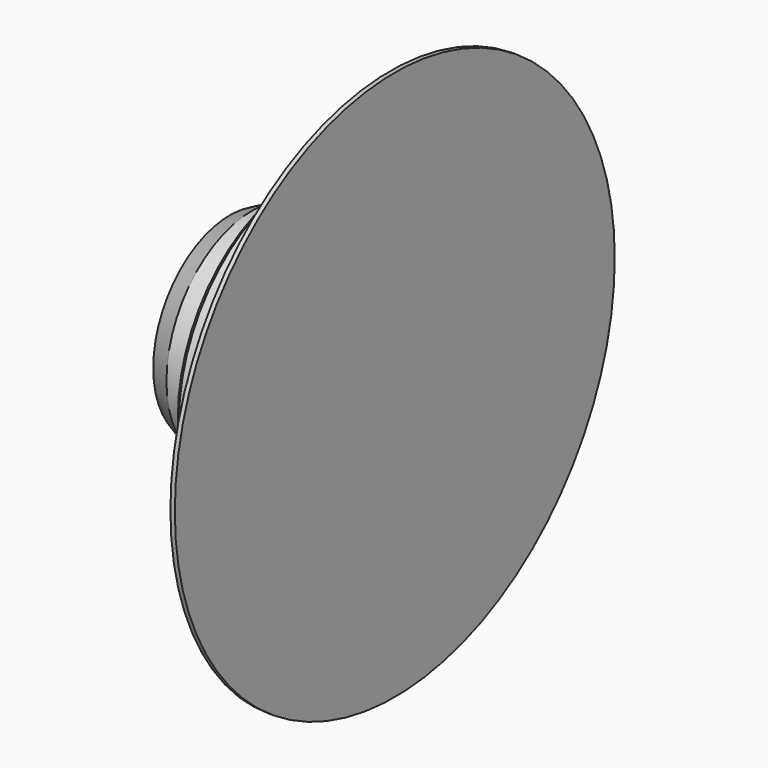
from build123d import *

# Parameters (mm, degrees)
F0_R       = 10
F1_DEPTH   = 4
F2_R       = 4.85
F3_DEPTH   = 3.5
F4_R       = 6.95
F4_R_2     = 6
F5_DEPTH   = 0.5
F6_R       = 10
F6_R_2     = 6.95
F7_DEPTH   = 3
F8_SIZE    = 0.25
F9_SIZE2   = 0.99999
F9_SIZE    = 0.49999
F9_2_SIZE2 = 1
F9_2_SIZE  = 0.5
F10_R      = 12.5
F10_R_2    = 9.5
F11_DEPTH  = 0.2


# Not quite as in the source:
# - a fillet or chamfer is up to 0.001 mm smaller than in the source, because OpenCascade refuses the exact size


with BuildPart() as f1:
    # F0 (on Right) → F1 (new body)
    with BuildSketch(Plane.YZ):
        Circle(F0_R)
    extrude(amount=F1_DEPTH)

    # F2 (on face) → F3 (join)
    with BuildSketch(Plane(origin=(0, 0, 0), x_dir=(0, -1, 0), z_dir=(-1, 0, 0))):
        Circle(F2_R)
    extrude(amount=F3_DEPTH)

    # F4 (on face) → F5 (join)
    with BuildSketch(Plane(origin=(0, 0, 0), x_dir=(0, -1, 0), z_dir=(-1, 0, 0))):
        Circle(F4_R)
        Circle(F4_R_2, mode=Mode.SUBTRACT)
    extrude(amount=F5_DEPTH)

    # F6 (on face) → F7 (cut)
    with BuildSketch(Plane(origin=(0, 0, 0), x_dir=(0, -1, 0), z_dir=(-1, 0, 0))):
        Circle(F6_R)
        Circle(F6_R_2, mode=Mode.SUBTRACT)
    extrude(amount=-F7_DEPTH, mode=Mode.SUBTRACT)

    # F8
    f8_edges = [f1.edges().sort_by_distance(p)[0] for p in [
        (-0.5, 6.95, 0),
        (-0.5, 6, 0),
    ]]
    chamfer(f8_edges, length=F8_SIZE)

    # F9 (size 0.5 and 1 in the source; OpenCascade refuses exactly that, so slightly less here)
    f9_edges = [f1.edges().sort_by_distance(p)[0] for p in [
        (4, -10, 0),
    ]]
    f9_side = f1.faces().sort_by_distance((4, 0, 0))[0]
    chamfer(f9_edges, length=F9_SIZE, length2=F9_SIZE2, reference=f9_side)

    # F9#2
    f9_2_edges = [f1.edges().sort_by_distance(p)[0] for p in [
        (-3.5, 4.85, 0),
    ]]
    f9_2_side = f1.faces().sort_by_distance((-3.5, 0, 0))[0]
    chamfer(f9_2_edges, length=F9_2_SIZE, length2=F9_2_SIZE2, reference=f9_2_side)

    # F10 (on face) → F11 (join)
    with BuildSketch(Plane.YZ.offset(4)):
        Circle(F10_R)
        Circle(F10_R_2, mode=Mode.SUBTRACT)
    extrude(amount=-F11_DEPTH)


solid = f1.part
